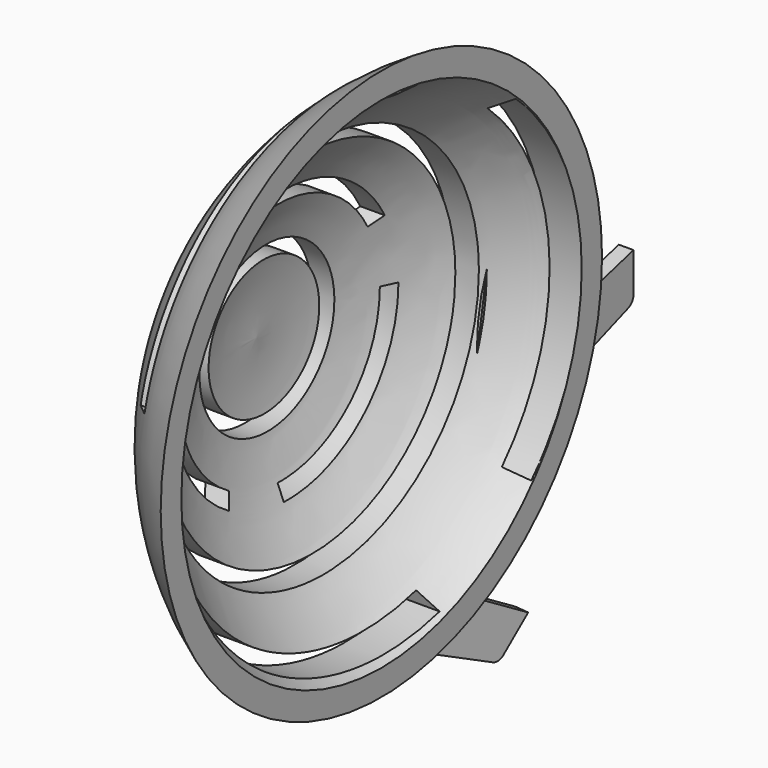
from build123d import *

# Parameters (mm, degrees)
F0_R      = 55.6269780277
F1_DEPTH  = 30
F6_R      = 39.2000488422
F6_R_2    = 36.2000488422
F6_R_3    = 16.8636065264
F6_R_4    = 13.8636065264
F7_DEPTH  = 100
F8_DEPTH  = 3
F9_ANGLE  = 7.9037236007
F11_ANGLE = 45


# Not quite as in the source:
# - a fillet or chamfer that OpenCascade refuses, or shapes differently, is made with other operations: its cross-section is extruded or revolved along the edge and cut away or added


with BuildPart() as f1:
    # F0 (on Right) → F1 (new body)
    with BuildSketch(Plane.YZ):
        with Locations((-56.2660247087, 47.6318523288)):
            Circle(F0_R)
    extrude(amount=F1_DEPTH)

    # F2: fillet of radius 55 on 1 edges, made by hand

    # F2_s1 → F2_t2 (revolve, cut)
    with BuildSketch(Plane.XY.offset(47.6318523288)):
        with BuildLine():
            ThreePointArc((55, -0.639046681), (16.1091270347, -16.7481737158), (0, -55.639046681))
            Line((0, -55.639046681), (0, -0.639046681))
            Line((0, -0.639046681), (55, -0.639046681))
        make_face()
    revolve(axis=Axis((0, -56.2660247087, 47.6318523288), (1, 0, 0)), mode=Mode.SUBTRACT)


with BuildPart() as f4:
    # F3 (on Top) → F4 (revolve)
    with BuildSketch(Plane.XY):
        with BuildLine():
            Line((28.9836188731, 69.3710569376), (24.4717162848, 69.3710569376))
            ThreePointArc((24.4717162848, 69.3710569376), (31.3874078401, 36.9410291189), (54.4717162848, 13.1366556207))
            Line((54.4717162848, 13.1366556207), (54.4717162848, 18.3955469453))
            ThreePointArc((54.4717162848, 18.3955469453), (34.6847571867, 40.3617994363), (28.9836188731, 69.3710569376))
        make_face()
    revolve(axis=Axis((39.4717162848, 69.3710569376, 0), (1, 0, 0)))

    # F6 (on Right) → F7 (cut)
    with BuildSketch(Plane.YZ):
        with BuildLine():
            ThreePointArc((107.9099874375, -33.0941581178), (120.3581686932, 2.6723928594), (104.1632820501, 36.9058418822))
            Line((104.1632820501, 36.9058418822), (102.1392633234, 34.6914913693))
            ThreePointArc((102.1392633234, 34.6914913693), (117.3624567679, 2.5120492878), (105.6611663876, -31.1085086307))
            Line((105.6611663876, -31.1085086307), (107.9099874375, -33.0941581178))
        make_face()
        with BuildLine():
            ThreePointArc((23.0511198621, -15.9773637116), (47.7787625663, -44.5750816629), (85.4562341901, -47.6885873668))
            Line((85.4562341901, -47.6885873668), (84.554638335, -44.8272721248))
            ThreePointArc((84.554638335, -44.8272721248), (49.1378150087, -41.9005767631), (25.8938308667, -15.0187218889))
            Line((25.8938308667, -15.0187218889), (23.0511198621, -15.9773637116))
        make_face()
        with BuildLine():
            ThreePointArc((80.2143225732, 49.0332532117), (43.0940228108, 41.8660270202), (21.6018847449, 10.7633938988))
            Line((21.6018847449, 10.7633938988), (24.5315498566, 10.1175902648))
            ThreePointArc((24.5315498566, 10.1175902648), (44.7341596385, 39.354065399), (79.6272414151, 46.091258019))
            Line((79.6272414151, 46.091258019), (80.2143225732, 49.0332532117))
        make_face()
        with Locations((70.4296366057, 0)):
            Circle(F6_R)
        with Locations((70.4296366057, 0)):
            Circle(F6_R_2, mode=Mode.SUBTRACT)
        with BuildLine():
            ThreePointArc((46.5782481819, 14.666672092), (43.2609475985, -6.7721737742), (56.2527821449, -24.1457407755))
            Line((56.2527821449, -24.1457407755), (57.7717308372, -21.558697121))
            ThreePointArc((57.7717308372, -21.558697121), (46.1718785635, -6.0465837269), (49.1337540844, 13.0952429393))
            Line((49.1337540844, 13.0952429393), (46.5782481819, 14.666672092))
        make_face()
        with Locations((70.4296366057, 0)):
            Circle(F6_R_3)
        with Locations((70.4296366057, 0)):
            Circle(F6_R_4, mode=Mode.SUBTRACT)
        with BuildLine():
            ThreePointArc((95.00819082, 13.4124819752), (78.050697035, 26.9428921598), (56.5183448775, 24.2997111598))
            Line((56.5183448775, 24.2997111598), (58.0088404198, 21.6961706784))
            ThreePointArc((58.0088404198, 21.6961706784), (77.2341548461, 24.0561537141), (92.3747742971, 11.975430335))
            Line((92.3747742971, 11.975430335), (95.00819082, 13.4124819752))
        make_face()
        with BuildLine():
            Line((69.9194325241, -24.9947932937), (69.8582080343, -27.994168489))
            ThreePointArc((69.8582080343, -27.994168489), (90.025554548, -20), (98.4296366057, 0))
            Line((98.4296366057, 0), (95.4296366057, 0))
            ThreePointArc((95.4296366057, 0), (87.9259919113, -17.8571428571), (69.9194325241, -24.9947932937))
        make_face()
    extrude(amount=F7_DEPTH, mode=Mode.SUBTRACT)


with BuildPart() as f8:
    # F5 (on Right) → F8 (new body)
    with BuildSketch(Plane.YZ):
        with BuildLine():
            Line((134.9051892757, 10.9073808417), (130.6237131357, -13.5129224509))
            Line((130.6237131357, -13.5129224509), (143.3325441838, -23.9233472419))
            ThreePointArc((143.3325441838, -23.9233472419), (145.6563583881, -24.9835409237), (148.2005874438, -24.7576612866))
            Line((148.2005874438, -24.7576612866), (169.87256579, -16.9244172467))
            ThreePointArc((169.87256579, -16.9244172467), (170.8297435306, -16.1924902765), (171.1927201099, -15.04351059))
            Line((171.1927201099, -15.04351059), (171.1927201099, -7.0412634909))
            Line((171.1927201099, -7.0412634909), (152.7985268051, -11.9345142706))
            ThreePointArc((152.7985268051, -11.9345142706), (149.6320549884, -11.7352286085), (147.2229963574, -9.6705990888))
            Line((147.2229963574, -9.6705990888), (134.9051892757, 10.9073808417))
        make_face()
    extrude(amount=F8_DEPTH)


with BuildPart() as f8b:
    # F5 (on Right) → F8, piece 2 (new body)
    with BuildSketch(Plane.YZ):
        with BuildLine():
            Line((142.6771916623, 126.3134279201), (138.3957155223, 101.8931246276))
            Line((138.3957155223, 101.8931246276), (151.1045465704, 91.4826998365))
            ThreePointArc((151.1045465704, 91.4826998365), (153.4283607746, 90.4225061548), (155.9725898304, 90.6483857919))
            Line((155.9725898304, 90.6483857919), (177.6445681765, 98.4816298317))
            ThreePointArc((177.6445681765, 98.4816298317), (178.6017459172, 99.213556802), (178.9647224964, 100.3625364884))
            Line((178.9647224964, 100.3625364884), (178.9647224964, 108.3647835876))
            Line((178.9647224964, 108.3647835876), (160.5705291917, 103.4715328079))
            ThreePointArc((160.5705291917, 103.4715328079), (157.404057375, 103.67081847), (154.9949987439, 105.7354479896))
            Line((154.9949987439, 105.7354479896), (142.6771916623, 126.3134279201))
        make_face()
    extrude(amount=F8_DEPTH)


with BuildPart() as f8_1:
    # F9: moved
    add(f8.part.rotate(Axis((0, 132.7644512057, -1.3027708046), (0, -0.1726903985, -0.9849761552)), F9_ANGLE))


with BuildPart() as f8_2:
    # F10: moved
    add(f8_1.part.moved(Location((38.4, -25.9, -53))))


with BuildPart() as f8_3:
    # F11: moved
    add(f8_2.part.rotate(Axis((39.8857507931, 108.8020247676, -42.0569994535), (-0.9905005288, 0.1354430054, -0.0237464699)), F11_ANGLE))


with BuildPart() as f8_4:
    # F12: moved
    add(f8_3.part.moved(Location((1.4, -3.3, 16.6))))


with BuildPart() as f8b_1:
    # F13: moved
    add(f8b.part.moved(Location((40, -31, -120))))


solid = Compound([f4.part, f8_4.part, f8b_1.part])
